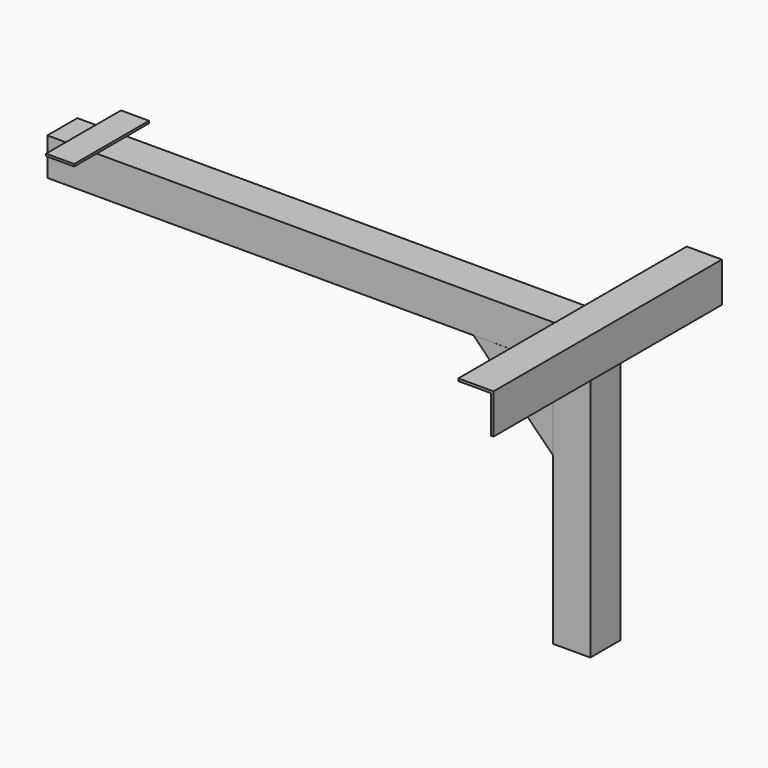
from build123d import *

# Parameters (mm, degrees)
F0_W      = 50.8
F0_H      = 387.35
F1_DEPTH  = 6.35
F2_W      = 6.35
F2_H      = 387.35
F3_DEPTH  = 50.8
F4_DEPTH  = 3.048
F5_DEPTH  = 3.048
F6_W      = 692.15
F6_H      = 50.8
F7_DEPTH  = 50.8
F8_W      = 38.1
F8_H      = 50.8
F8_H_2    = 38.1
F9_DEPTH  = 3.048
F10_W     = 50.8
F10_H     = 50.8
F11_DEPTH = 333.375
F13_DEPTH = 50.8


# Not quite as in the source:
# - a feature names something its author has since deleted; it is built from what else it names


with BuildPart() as f1:
    # F0 (on Top) → F1 (new body)
    with BuildSketch(Plane.XY):
        Rectangle(F0_W, F0_H)
    extrude(amount=F1_DEPTH)

    # F2 (on face) → F3 (join)
    with BuildSketch(Plane(origin=(0, 0, 0), x_dir=(1, 0, 0), z_dir=(0, 0, -1))):
        with Locations((22.225, 0)):
            Rectangle(F2_W, F2_H)
    extrude(amount=F3_DEPTH)

    # F4 (cut): a face of the model
    f4_faces = [f1.faces().sort_by_distance(p)[0] for p in [
        (25.4, 0, -22.225),
    ]]
    extrude(f4_faces, amount=-F4_DEPTH, mode=Mode.SUBTRACT)

    # F5 (cut): a face of the model
    f5_faces = [f1.faces().sort_by_distance(p)[0] for p in [
        (-1.524, 0, 6.35),
    ]]
    extrude(f5_faces, amount=-F5_DEPTH, mode=Mode.SUBTRACT)

    # F6 (on face) → F7 (join)
    with BuildSketch(Plane(origin=(0, 0, 0), x_dir=(1, 0, 0), z_dir=(0, 0, -1))):
        Polygon((19.05, -25.4), (19.05, 0), (19.05, 25.4), (-25.4, 25.4), (-25.4, -25.4), align=None)
        with Locations((-371.475, 0)):
            Rectangle(F6_W, F6_H)
    extrude(amount=F7_DEPTH)

    # F8 (on face) → F9 (join)
    with BuildSketch(Plane.XY):
        with Locations((-669.798, 0)):
            Rectangle(F8_W, F8_H)
        with Locations((-669.798, 44.45)):
            Rectangle(F8_W, F8_H_2)
        with Locations((-669.798, -44.45)):
            Rectangle(F8_W, F8_H_2)
    extrude(amount=F9_DEPTH)

    # F10 (on face) → F11 (join)
    with BuildSketch(Plane(origin=(0, 0, -50.8), x_dir=(1, 0, 0), z_dir=(0, 0, -1))):
        with Locations((-6.35, 0)):
            Rectangle(F10_W, F10_H)
    extrude(amount=F11_DEPTH)


with BuildPart() as f13:
    # F12 (on face) → F13 (new body)
    with BuildSketch(Plane.XZ.offset(25.4)):
        Polygon((-67.7644877579, -50.8934632736), (-139.7, -50.8), (-31.75, -158.75), (-31.75, -86.9079510314), (-49.8039755157, -68.8539755157), align=None)
    extrude(amount=-F13_DEPTH)


solid = Compound([f1.part, f13.part])
